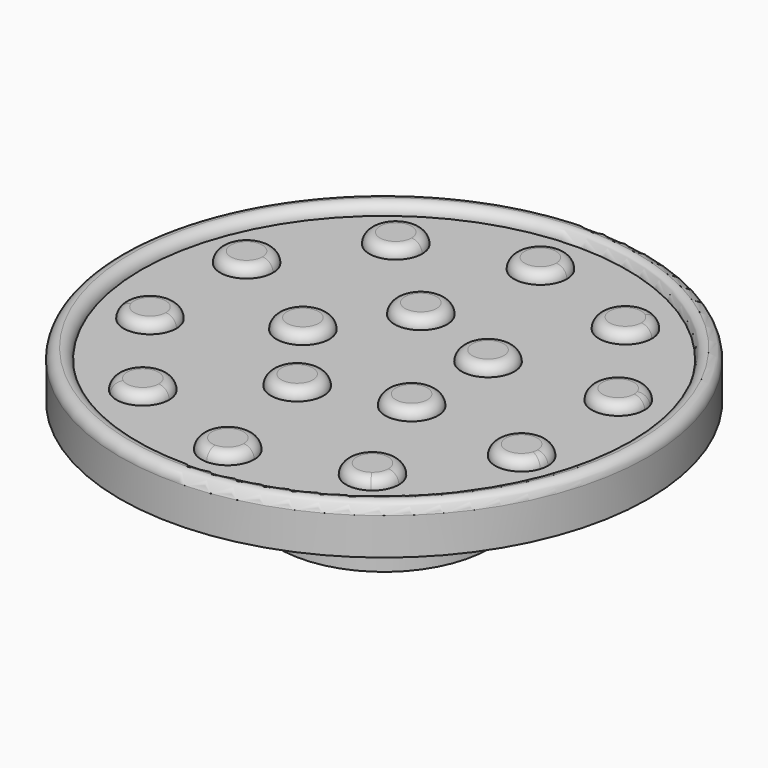
from build123d import *

# Parameters (mm, degrees)
F0_R     = 10
F0_R_2   = 4
F1_DEPTH = 1.4
F2_DEPTH = 5
F3_R     = 10
F3_R_2   = 9.2
F3_R_3   = 1
F4_DEPTH = 0.4
F5_R     = 0.39999


# Not quite as in the source:
# - a fillet or chamfer is up to 0.001 mm smaller than in the source, because OpenCascade refuses the exact size


with BuildPart() as f1:
    # F0 (on Top) → F1 (new body)
    with BuildSketch(Plane.XY):
        with Locations((-37.5053957105, 22.3950315267)):
            Circle(F0_R)
        with Locations((-37.5053957105, 22.3950315267)):
            Circle(F0_R_2, mode=Mode.SUBTRACT)
        with Locations((-37.5053957105, 22.3950315267)):
            Circle(F0_R_2)
    extrude(amount=-F1_DEPTH)

    # F0 (on Top) → F2 (join)
    with BuildSketch(Plane.XY):
        with Locations((-37.5053957105, 22.3950315267)):
            Circle(F0_R_2)
    extrude(amount=-F2_DEPTH)

    # F3 (on face) → F4 (join)
    with BuildSketch(Plane.XY):
        with Locations((-37.5053957105, 22.3950315267)):
            Circle(F3_R)
        with Locations((-37.5053957105, 22.3950315267)):
            Circle(F3_R_2, mode=Mode.SUBTRACT)
        with BuildLine():
            ThreePointArc((-43.5432139311, 24.6817572851), (-44.3867794879, 25.6694456291), (-45.4942704611, 24.9907742372))
            ThreePointArc((-45.4942704611, 24.9907742372), (-44.6996483742, 23.694068941), (-43.5432139311, 24.6817572851))
        make_face()
        with BuildLine():
            ThreePointArc((-43.5432139311, 20.1083057683), (-44.6996483831, 21.095994111), (-45.4942704555, 19.799288799))
            ThreePointArc((-45.4942704555, 19.799288799), (-44.386779479, 19.1206174257), (-43.5432139311, 20.1083057683))
        make_face()
        with BuildLine():
            ThreePointArc((-40.8550065774, 16.4083057683), (-42.3089970383, 17.2993123123), (-42.4427919004, 15.5992888253))
            ThreePointArc((-42.4427919004, 15.5992888253), (-41.4010161166, 15.5172992243), (-40.8550065774, 16.4083057683))
        make_face()
        with BuildLine():
            ThreePointArc((-37.5053957105, 30.7950315267), (-38.2125024917, 29.0879247455), (-36.5053957105, 29.7950315267))
            ThreePointArc((-36.5053957105, 29.7950315267), (-36.7982889293, 30.5021383079), (-37.5053957105, 30.7950315267))
        make_face()
        with BuildLine():
            ThreePointArc((-40.8550065774, 28.3817572851), (-41.4010160436, 29.2727637919), (-42.4427917678, 29.1907743244))
            ThreePointArc((-42.4427917678, 29.1907743244), (-42.3089971113, 27.4907507782), (-40.8550065774, 28.3817572851))
        make_face()
        with BuildLine():
            ThreePointArc((-36.5053957105, 14.9950315267), (-38.2125024917, 15.7021383079), (-37.5053957105, 13.9950315267))
            ThreePointArc((-37.5053957105, 13.9950315267), (-36.7982889293, 14.2879247455), (-36.5053957105, 14.9950315267))
        make_face()
        with BuildLine():
            ThreePointArc((-32.1557848435, 16.4083057683), (-34.0467913678, 16.8622962678), (-32.5679995907, 15.5992887743))
            ThreePointArc((-32.5679995907, 15.5992887743), (-32.2647783192, 15.9543152688), (-32.1557848435, 16.4083057683))
        make_face()
        with BuildLine():
            ThreePointArc((-29.4675774899, 20.1083057683), (-31.4552658317, 20.2647402258), (-29.5165209689, 19.7992887885))
            ThreePointArc((-29.5165209689, 19.7992887885), (-29.4798891481, 19.9518713108), (-29.4675774899, 20.1083057683))
        make_face()
        with BuildLine():
            ThreePointArc((-29.4675774899, 24.6817572851), (-29.4798891518, 24.8381917658), (-29.5165209834, 24.9907743097))
            ThreePointArc((-29.5165209834, 24.9907743097), (-31.455265828, 24.5253228043), (-29.4675774899, 24.6817572851))
        make_face()
        with BuildLine():
            ThreePointArc((-32.1557848435, 28.3817572851), (-32.2647783192, 28.8357477845), (-32.5679995907, 29.1907742791))
            ThreePointArc((-32.5679995907, 29.1907742791), (-34.0467913678, 27.9277667856), (-32.1557848435, 28.3817572851))
        make_face()
        with Locations((-38.4562697482, 25.3215208985)):
            Circle(F3_R_3)
        with Locations((-40.5824887346, 22.3950315267)):
            Circle(F3_R_3)
        with Locations((-38.4562697482, 19.4685421549)):
            Circle(F3_R_3)
        with Locations((-35.0159751607, 20.5863616272)):
            Circle(F3_R_3)
        with Locations((-35.0159751607, 24.2037014262)):
            Circle(F3_R_3)
    extrude(amount=F4_DEPTH)

    # F5 (radius 0.4 in the source; OpenCascade refuses exactly that, so slightly less here)
    f5_edges = [f1.edges().sort_by_distance(p)[0] for p in [
        (-43.592157, 24.37274, 0.4),
        (-43.592157, 20.417323, 0.4),
        (-41.267221, 17.217323, 0.4),
        (-39.45627, 19.468542, 0.4),
        (-41.582489, 22.395032, 0.4),
        (-36.015975, 20.586362, 0.4),
        (-37.505396, 15.995032, 0.4),
        (-33.74357, 17.217323, 0.4),
        (-31.418634, 20.417323, 0.4),
        (-31.418634, 24.37274, 0.4),
        (-36.015975, 24.203701, 0.4),
        (-39.45627, 25.321521, 0.4),
        (-41.267221, 27.57274, 0.4),
        (-38.505396, 29.795032, 0.4),
        (-33.74357, 27.57274, 0.4),
        (-46.705396, 22.395032, 0.4),
        (-47.505396, 22.395032, 0.4),
    ]]
    fillet(f5_edges, radius=F5_R)


solid = f1.part
